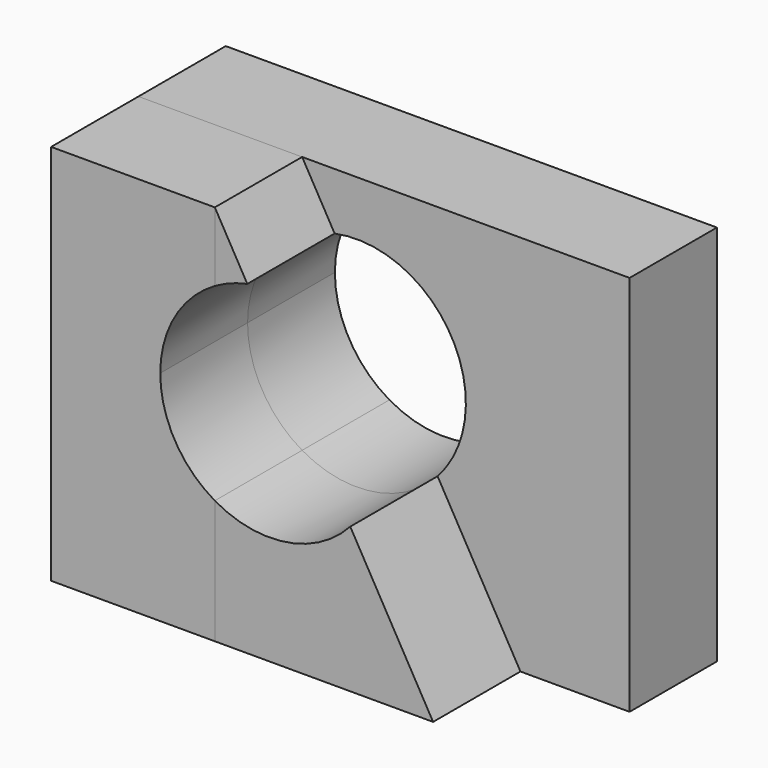
from build123d import *

# Parameters (mm, degrees)
F0_W     = 57.15
F0_H     = 44.45
F1_DEPTH = 12.7
F2_W     = 19.05
F2_H     = 12.7
F3_DEPTH = 44.45
F5_DEPTH = 12.7
F7_DEPTH = 25.4


# Not quite as in the source:
# - a feature of the source that left no trace in its solid (it failed there, or was rolled back) is left out


with BuildPart() as f1:
    # F0 (on Front) → F1 (new body)
    with BuildSketch(Plane.XZ):
        with Locations((28.575, 22.225)):
            Rectangle(F0_W, F0_H)
    extrude(amount=F1_DEPTH)


with BuildPart() as f3:
    # F2 (on face) → F3 (new body)
    with BuildSketch(Plane.XY.offset(44.45)):
        with Locations((9.525, -19.05)):
            Rectangle(F2_W, F2_H)
    extrude(amount=-F3_DEPTH)


with BuildPart() as f5:
    # F4 (on face) → F5 (new body)
    with BuildSketch(Plane.XZ.offset(12.7)):
        Polygon((44.45, 0), (19.05, 44.45), (19.05, 0), align=None)
    extrude(amount=F5_DEPTH)


with BuildPart() as f7_tool:
    # F6 (on face) → F7 (new body)
    with BuildSketch(Plane(origin=(0, 0, 0), x_dir=(-1, 0, 0), z_dir=(0, 1, 0))):
        with BuildLine():
            ThreePointArc((-22.8288518953, 37.8370091832), (-36.426687905, 31.7009645171), (-34.8096096432, 16.8706831245))
            Line((-34.8096096432, 16.8706831245), (-22.8288518953, 37.8370091832))
        make_face()
        with BuildLine():
            Line((-22.8288518953, 37.8370091832), (-34.8096096432, 16.8706831245))
            ThreePointArc((-34.8096096432, 16.8706831245), (-27.3658451247, 12.8530699792), (-19.05, 14.4014773719))
            Line((-19.05, 14.4014773719), (-19.05, 36.3985226281))
            ThreePointArc((-19.05, 36.3985226281), (-20.8818110078, 37.2691182584), (-22.8288518953, 37.8370091832))
        make_face()
        with BuildLine():
            Line((-19.05, 36.3985226281), (-19.05, 14.4014773719))
            ThreePointArc((-19.05, 14.4014773719), (-14.4014773719, 19.05), (-12.7, 25.4))
            ThreePointArc((-12.7, 25.4), (-14.4014773719, 31.75), (-19.05, 36.3985226281))
        make_face()
    extrude(amount=-F7_DEPTH)


with BuildPart() as f1_1:
    add(f1.part)

    # F7: cut by f7_tool
    add(f7_tool.part, mode=Mode.SUBTRACT)


with BuildPart() as f3_1:
    add(f3.part)

    # F7: cut by f7_tool
    add(f7_tool.part, mode=Mode.SUBTRACT)


with BuildPart() as f5_1:
    add(f5.part)

    # F7: cut by f7_tool
    add(f7_tool.part, mode=Mode.SUBTRACT)


solid = Compound([f1_1.part, f3_1.part, f5_1.part])
